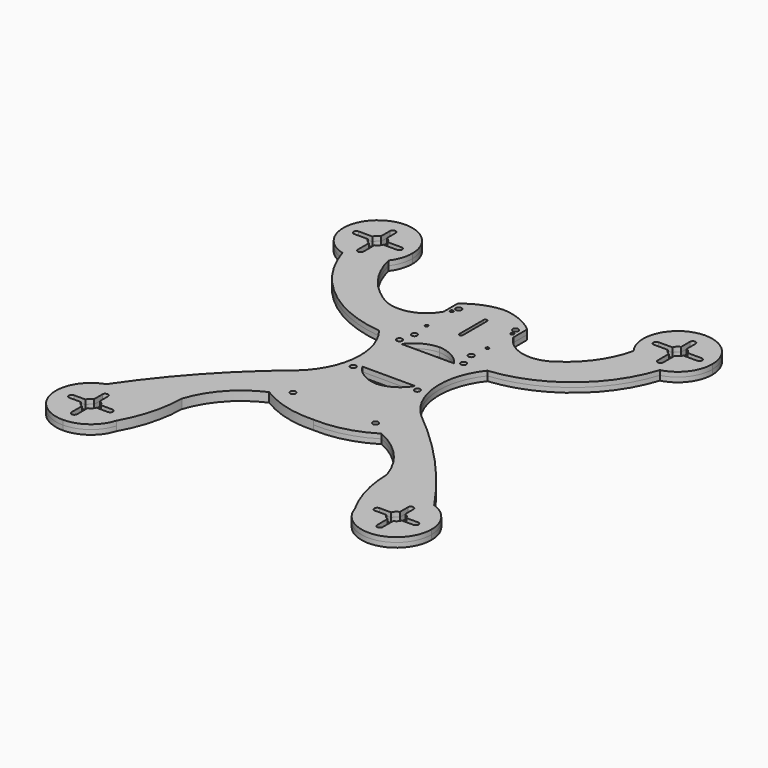
from build123d import *

# Parameters (mm, degrees)
F0_R     = 1.51
F0_R_2   = 1.5
F0_R_3   = 0.8286154485
F1_DEPTH = 2.5


# Not quite as in the source:
# - a feature names something its author has since deleted; it is built from what else it names


with BuildPart() as f1:
    # F0 (on Top) → F1 (new body, symmetric)
    with BuildSketch(Plane.XY):
        with BuildLine():
            Line((-30.1874730734, -52.384633545), (0, -52.384633545))
            Line((0, -52.384633545), (30.1874730734, -52.384633545))
            ThreePointArc((30.1874730734, -52.384633545), (45.5377526982, -63.4637920797), (55.0844569757, -79.8112468001))
            ThreePointArc((55.0844569757, -79.8112468001), (57.4877299486, -96.795391674), (64.006494816, -112.6617902157))
            ThreePointArc((64.006494816, -112.6617902157), (68.9048734281, -93.7156261949), (87.9887831434, -89.3848486541))
            ThreePointArc((87.9887831434, -89.3848486541), (62.7573722568, -57.4704416031), (33.2118480486, -29.5023263287))
            ThreePointArc((33.2118480486, -29.5023263287), (26.7242341229, -24.347436704), (20.0885272052, -19.384633545))
            Line((20.0885272052, -19.384633545), (21.4383106123, 19.6198565499))
            ThreePointArc((21.4383106123, 19.6198565499), (25.2461771825, 19.6733705963), (29.0445808108, 19.9469422451))
            ThreePointArc((29.0445808108, 19.9469422451), (63.9115542942, 34.3327431649), (85.1620762927, 65.494778124))
            ThreePointArc((85.1620762927, 65.494778124), (74.4508574846, 65.9052964442), (65.7591074705, 72.1784308553))
            ThreePointArc((65.7591074705, 72.1784308553), (58.8481462627, 56.5107805649), (46.674050137, 44.4680219955))
            ThreePointArc((46.674050137, 44.4680219955), (45.2140675367, 43.468299654), (43.6672608264, 42.60900753))
            ThreePointArc((43.6672608264, 42.60900753), (31.6040521188, 37.8807075534), (18.7, 36.713118625))
            Line((18.7, 36.713118625), (18.7, 50.3240376711))
            Line((18.7, 50.3240376711), (18.7, 59.615366455))
            ThreePointArc((18.7, 59.615366455), (9.9937787785, 65.0337535356), (0, 67.3319250345))
            ThreePointArc((0, 67.3319250345), (-9.9937787785, 65.0337535356), (-18.7, 59.615366455))
            Line((-18.7, 59.615366455), (-18.7, 50.3240376711))
            Line((-18.7, 50.3240376711), (-18.7, 36.713118625))
            ThreePointArc((-18.7, 36.713118625), (-31.6040521188, 37.8807075534), (-43.6672608264, 42.60900753))
            ThreePointArc((-43.6672608264, 42.60900753), (-45.2140675367, 43.468299654), (-46.674050137, 44.4680219955))
            ThreePointArc((-46.674050137, 44.4680219955), (-58.8481462627, 56.5107805649), (-65.7591074705, 72.1784308553))
            ThreePointArc((-65.7591074705, 72.1784308553), (-74.4508574846, 65.9052964442), (-85.1620762927, 65.494778124))
            ThreePointArc((-85.1620762927, 65.494778124), (-63.9115542942, 34.3327431649), (-29.0445808108, 19.9469422451))
            ThreePointArc((-29.0445808108, 19.9469422451), (-25.2461771825, 19.6733705963), (-21.4383106123, 19.6198565499))
            Line((-21.4383106123, 19.6198565499), (-20.0885272052, -19.384633545))
            ThreePointArc((-20.0885272052, -19.384633545), (-26.7242341229, -24.347436704), (-33.2118480486, -29.5023263287))
            ThreePointArc((-33.2118480486, -29.5023263287), (-62.7573722568, -57.4704416031), (-87.9887831434, -89.3848486541))
            ThreePointArc((-87.9887831434, -89.3848486541), (-71.0247151945, -91.9413319507), (-63.1980110774, -107.2075662893))
            ThreePointArc((-63.1980110774, -107.2075662893), (-63.4012302478, -109.9644759992), (-64.006494816, -112.6617902157))
            ThreePointArc((-64.006494816, -112.6617902157), (-57.4877299486, -96.795391674), (-55.0844569757, -79.8112468001))
            ThreePointArc((-55.0844569757, -79.8112468001), (-45.5377526982, -63.4637920797), (-30.1874730734, -52.384633545))
        make_face()
        with Locations((-22.1585966647, -46.4437194169)):
            Circle(F0_R, mode=Mode.SUBTRACT)
        with Locations((-17.2166451812, -12.1963914914)):
            Circle(F0_R_2, mode=Mode.SUBTRACT)
        with Locations((22.1585966647, -46.4437194169)):
            Circle(F0_R, mode=Mode.SUBTRACT)
        with BuildLine():
            Line((-14.1357257962, -9.8804375157), (0, -9.8804375157))
            Line((0, -9.8804375157), (14.1357257962, -9.8804375157))
            ThreePointArc((14.1357257962, -9.8804375157), (8.1506579233, -15.9532697198), (0, -18.4566881508))
            ThreePointArc((0, -18.4566881508), (-8.1506579233, -15.9532697198), (-14.1357257962, -9.8804375157))
        make_face(mode=Mode.SUBTRACT)
        with Locations((17.2166451812, -12.1963914914)):
            Circle(F0_R_2, mode=Mode.SUBTRACT)
        with BuildLine():
            ThreePointArc((-18.7, 18.5807666779), (-18.7166451812, 18.8036085086), (-18.7, 19.0264503392))
            ThreePointArc((-18.7, 19.0264503392), (-17.1049138701, 20.2994414251), (-15.7166451812, 18.8036085086))
            ThreePointArc((-15.7166451812, 18.8036085086), (-17.1049138701, 17.3077755921), (-18.7, 18.5807666779))
        make_face(mode=Mode.SUBTRACT)
        with Locations((-15.2508411556, 26.3805482537)):
            Circle(F0_R, mode=Mode.SUBTRACT)
        with Locations((-16.3033773307, 35.8986854553)):
            Circle(F0_R_3, mode=Mode.SUBTRACT)
        with BuildLine():
            ThreePointArc((-17.2290705489, 52.7536339848), (-16.3040705489, 53.6786339848), (-15.3790705489, 52.7536339848))
            ThreePointArc((-15.3790705489, 52.7536339848), (-16.3040705489, 51.8286339848), (-17.2290705489, 52.7536339848))
        make_face(mode=Mode.SUBTRACT)
        with Locations((-15.2508411556, 56.1236590147)):
            Circle(F0_R, mode=Mode.SUBTRACT)
        with BuildLine():
            ThreePointArc((-14.1357257962, 16.3518823683), (-7.9488995039, 21.8256144878), (0, 24.0736268461))
            ThreePointArc((0, 24.0736268461), (7.9488995039, 21.8256144878), (14.1357257962, 16.3518823683))
            Line((14.1357257962, 16.3518823683), (0, 16.3518823683))
            Line((0, 16.3518823683), (-14.1357257962, 16.3518823683))
        make_face(mode=Mode.SUBTRACT)
        with Locations((15.2508411556, 26.3805482537)):
            Circle(F0_R, mode=Mode.SUBTRACT)
        with BuildLine():
            ThreePointArc((18.7, 18.5807666779), (15.7166451812, 18.8036085086), (18.7, 19.0264503392))
            ThreePointArc((18.7, 19.0264503392), (18.7124780977, 18.9153398197), (18.7166451812, 18.8036085086))
            ThreePointArc((18.7166451812, 18.8036085086), (18.7124780977, 18.6918771974), (18.7, 18.5807666779))
        make_face(mode=Mode.SUBTRACT)
        with Locations((16.3033773307, 35.8986854553)):
            Circle(F0_R_3, mode=Mode.SUBTRACT)
        with BuildLine():
            ThreePointArc((0.925, 38.6986881495), (0.6540737726, 38.0446143769), (0, 37.7736881495))
            ThreePointArc((0, 37.7736881495), (-0.6540737726, 38.0446143769), (-0.925, 38.6986881495))
            Line((-0.925, 38.6986881495), (-0.925, 54.8593327403))
            ThreePointArc((-0.925, 54.8593327403), (-0.6540737726, 55.5134065129), (0, 55.7843327403))
            ThreePointArc((0, 55.7843327403), (0.6540737726, 55.5134065129), (0.925, 54.8593327403))
            Line((0.925, 54.8593327403), (0.925, 38.6986881495))
        make_face(mode=Mode.SUBTRACT)
        with Locations((15.2508411556, 56.1236590147)):
            Circle(F0_R, mode=Mode.SUBTRACT)
        with BuildLine():
            ThreePointArc((15.3790705489, 52.7536339848), (16.3040705489, 53.6786339848), (17.2290705489, 52.7536339848))
            ThreePointArc((17.2290705489, 52.7536339848), (16.3040705489, 51.8286339848), (15.3790705489, 52.7536339848))
        make_face(mode=Mode.SUBTRACT)
        with BuildLine():
            ThreePointArc((-82, -126.0095552119), (-70.7981133375, -122.3083120538), (-64.006494816, -112.6617902157))
            ThreePointArc((-64.006494816, -112.6617902157), (-63.4012302478, -109.9644759992), (-63.1980110774, -107.2075662893))
            ThreePointArc((-63.1980110774, -107.2075662893), (-71.0247151945, -91.9413319507), (-87.9887831434, -89.3848486541))
            ThreePointArc((-87.9887831434, -89.3848486541), (-100.5555561355, -110.241725802), (-82, -126.0095552119))
        make_face()
        with BuildLine():
            ThreePointArc((-80.5, -103.1137172447), (-78.917014434, -104.1245807233), (-77.9061509554, -105.7075662893))
            Line((-77.9061509554, -105.7075662893), (-71.66, -105.7075662893))
            ThreePointArc((-71.66, -105.7075662893), (-70.5993398282, -106.1469061175), (-70.16, -107.2075662893))
            ThreePointArc((-70.16, -107.2075662893), (-70.5993398282, -108.2682264611), (-71.66, -108.7075662893))
            Line((-71.66, -108.7075662893), (-77.9061509554, -108.7075662893))
            ThreePointArc((-77.9061509554, -108.7075662893), (-78.917014434, -110.2905518553), (-80.5, -111.3014153339))
            Line((-80.5, -111.3014153339), (-80.5, -118.2955773668))
            ThreePointArc((-80.5, -118.2955773668), (-82, -119.7955773668), (-83.5, -118.2955773668))
            Line((-83.5, -118.2955773668), (-83.5, -111.3014153339))
            ThreePointArc((-83.5, -111.3014153339), (-85.082985566, -110.2905518553), (-86.0938490446, -108.7075662893))
            Line((-86.0938490446, -108.7075662893), (-92.34, -108.7075662893))
            ThreePointArc((-92.34, -108.7075662893), (-93.84, -107.2075662893), (-92.34, -105.7075662893))
            Line((-92.34, -105.7075662893), (-86.0938490446, -105.7075662893))
            ThreePointArc((-86.0938490446, -105.7075662893), (-85.082985566, -104.1245807233), (-83.5, -103.1137172447))
            Line((-83.5, -103.1137172447), (-83.5, -97.6055773668))
            ThreePointArc((-83.5, -97.6055773668), (-82, -96.1055773668), (-80.5, -97.6055773668))
            Line((-80.5, -97.6055773668), (-80.5, -103.1137172447))
        make_face(mode=Mode.SUBTRACT)
        with BuildLine():
            ThreePointArc((87.9887831434, -89.3848486541), (68.9048734281, -93.7156261949), (64.006494816, -112.6617902157))
            ThreePointArc((64.006494816, -112.6617902157), (84.7569097099, -125.8063360415), (100.8019889226, -107.2075662893))
            ThreePointArc((100.8019889226, -107.2075662893), (97.2662343387, -96.2322814839), (87.9887831434, -89.3848486541))
        make_face()
        with BuildLine():
            Line((83.5, -111.3014153339), (83.5, -118.2955773668))
            ThreePointArc((83.5, -118.2955773668), (82, -119.7955773668), (80.5, -118.2955773668))
            Line((80.5, -118.2955773668), (80.5, -111.3014153339))
            ThreePointArc((80.5, -111.3014153339), (78.917014434, -110.2905518553), (77.9061509554, -108.7075662893))
            Line((77.9061509554, -108.7075662893), (71.66, -108.7075662893))
            ThreePointArc((71.66, -108.7075662893), (70.16, -107.2075662893), (71.66, -105.7075662893))
            Line((71.66, -105.7075662893), (77.9061509554, -105.7075662893))
            ThreePointArc((77.9061509554, -105.7075662893), (78.917014434, -104.1245807233), (80.5, -103.1137172447))
            Line((80.5, -103.1137172447), (80.5, -97.6055773668))
            ThreePointArc((80.5, -97.6055773668), (82, -96.1055773668), (83.5, -97.6055773668))
            Line((83.5, -97.6055773668), (83.5, -103.1137172447))
            ThreePointArc((83.5, -103.1137172447), (85.082985566, -104.1245807233), (86.0938490446, -105.7075662893))
            Line((86.0938490446, -105.7075662893), (92.34, -105.7075662893))
            ThreePointArc((92.34, -105.7075662893), (93.4006601718, -106.1469061175), (93.84, -107.2075662893))
            ThreePointArc((93.84, -107.2075662893), (93.4006601718, -108.2682264611), (92.34, -108.7075662893))
            Line((92.34, -108.7075662893), (86.0938490446, -108.7075662893))
            ThreePointArc((86.0938490446, -108.7075662893), (85.082985566, -110.2905518553), (83.5, -111.3014153339))
        make_face(mode=Mode.SUBTRACT)
        with BuildLine():
            ThreePointArc((-61.9557945169, 83.4250120531), (-67.3831058615, 96.5277007085), (-80.4857945169, 101.9550120531))
            ThreePointArc((-80.4857945169, 101.9550120531), (-98.8652413898, 85.7823055534), (-85.1620762927, 65.494778124))
            ThreePointArc((-85.1620762927, 65.494778124), (-74.4508574846, 65.9052964442), (-65.7591074705, 72.1784308553))
            ThreePointArc((-65.7591074705, 72.1784308553), (-62.932355951, 77.4888774088), (-61.9557945169, 83.4250120531))
        make_face()
        with BuildLine():
            ThreePointArc((-78.9857945169, 87.5188610977), (-77.4028089509, 86.507997619), (-76.3919454723, 84.9250120531))
            Line((-76.3919454723, 84.9250120531), (-68.9257945169, 84.9250120531))
            ThreePointArc((-68.9257945169, 84.9250120531), (-67.8651343451, 84.4856722249), (-67.4257945169, 83.4250120531))
            ThreePointArc((-67.4257945169, 83.4250120531), (-67.8651343451, 82.3643518813), (-68.9257945169, 81.9250120531))
            Line((-68.9257945169, 81.9250120531), (-76.3919454723, 81.9250120531))
            ThreePointArc((-76.3919454723, 81.9250120531), (-77.4028089509, 80.3420264871), (-78.9857945169, 79.3311630085))
            Line((-78.9857945169, 79.3311630085), (-78.9857945169, 71.8650120531))
            ThreePointArc((-78.9857945169, 71.8650120531), (-80.4857945169, 70.3650120531), (-81.9857945169, 71.8650120531))
            Line((-81.9857945169, 71.8650120531), (-81.9857945169, 79.3311630085))
            ThreePointArc((-81.9857945169, 79.3311630085), (-83.5687800828, 80.3420264871), (-84.5796435615, 81.9250120531))
            Line((-84.5796435615, 81.9250120531), (-92.0457945169, 81.9250120531))
            ThreePointArc((-92.0457945169, 81.9250120531), (-93.5457945169, 83.4250120531), (-92.0457945169, 84.9250120531))
            Line((-92.0457945169, 84.9250120531), (-84.5796435615, 84.9250120531))
            ThreePointArc((-84.5796435615, 84.9250120531), (-83.5687800828, 86.507997619), (-81.9857945169, 87.5188610977))
            Line((-81.9857945169, 87.5188610977), (-81.9857945169, 93.4850120531))
            ThreePointArc((-81.9857945169, 93.4850120531), (-80.4857945169, 94.9850120531), (-78.9857945169, 93.4850120531))
            Line((-78.9857945169, 93.4850120531), (-78.9857945169, 87.5188610977))
        make_face(mode=Mode.SUBTRACT)
        with BuildLine():
            ThreePointArc((65.7591074705, 72.1784308553), (74.4508574846, 65.9052964442), (85.1620762927, 65.494778124))
            ThreePointArc((85.1620762927, 65.494778124), (95.1488842545, 72.0956387541), (99.0157945169, 83.4250120531))
            ThreePointArc((99.0157945169, 83.4250120531), (74.5496598725, 100.9784506189), (65.7591074705, 72.1784308553))
        make_face()
        with BuildLine():
            ThreePointArc((81.9857945169, 87.5188610977), (83.5687800828, 86.507997619), (84.5796435615, 84.9250120531))
            Line((84.5796435615, 84.9250120531), (92.0457945169, 84.9250120531))
            ThreePointArc((92.0457945169, 84.9250120531), (93.1064546886, 84.4856722249), (93.5457945169, 83.4250120531))
            ThreePointArc((93.5457945169, 83.4250120531), (93.1064546886, 82.3643518813), (92.0457945169, 81.9250120531))
            Line((92.0457945169, 81.9250120531), (84.5796435615, 81.9250120531))
            ThreePointArc((84.5796435615, 81.9250120531), (83.5687800828, 80.3420264871), (81.9857945169, 79.3311630085))
            Line((81.9857945169, 79.3311630085), (81.9857945169, 71.8650120531))
            ThreePointArc((81.9857945169, 71.8650120531), (80.4857945169, 70.3650120531), (78.9857945169, 71.8650120531))
            Line((78.9857945169, 71.8650120531), (78.9857945169, 79.3311630085))
            ThreePointArc((78.9857945169, 79.3311630085), (77.4028089509, 80.3420264871), (76.3919454723, 81.9250120531))
            Line((76.3919454723, 81.9250120531), (68.9257945169, 81.9250120531))
            ThreePointArc((68.9257945169, 81.9250120531), (67.4257945169, 83.4250120531), (68.9257945169, 84.9250120531))
            Line((68.9257945169, 84.9250120531), (76.3919454723, 84.9250120531))
            ThreePointArc((76.3919454723, 84.9250120531), (77.4028089509, 86.507997619), (78.9857945169, 87.5188610977))
            Line((78.9857945169, 87.5188610977), (78.9857945169, 93.4850120531))
            ThreePointArc((78.9857945169, 93.4850120531), (80.4857945169, 94.9850120531), (81.9857945169, 93.4850120531))
            Line((81.9857945169, 93.4850120531), (81.9857945169, 87.5188610977))
        make_face(mode=Mode.SUBTRACT)
        with BuildLine():
            Line((30.1874730734, -52.384633545), (0, -52.384633545))
            Line((0, -52.384633545), (-30.1874730734, -52.384633545))
            ThreePointArc((-30.1874730734, -52.384633545), (-15.6968009353, -58.6423760096), (0, -60.3004954755))
            ThreePointArc((0, -60.3004954755), (15.6968009353, -58.6423760096), (30.1874730734, -52.384633545))
        make_face()
        with BuildLine():
            ThreePointArc((-29.0445808108, 19.9469422451), (-21.3446813988, -5.6021854639), (-33.2118480486, -29.5023263287))
            ThreePointArc((-33.2118480486, -29.5023263287), (-26.7242341229, -24.347436704), (-20.0885272052, -19.384633545))
            Line((-20.0885272052, -19.384633545), (-21.4383106123, 19.6198565499))
            ThreePointArc((-21.4383106123, 19.6198565499), (-25.2461771825, 19.6733705963), (-29.0445808108, 19.9469422451))
        make_face()
        with BuildLine():
            ThreePointArc((20.0885272052, -19.384633545), (26.7242341229, -24.347436704), (33.2118480486, -29.5023263287))
            ThreePointArc((33.2118480486, -29.5023263287), (21.3446813988, -5.6021854639), (29.0445808108, 19.9469422451))
            ThreePointArc((29.0445808108, 19.9469422451), (25.2461771825, 19.6733705963), (21.4383106123, 19.6198565499))
            Line((21.4383106123, 19.6198565499), (20.0885272052, -19.384633545))
        make_face()
        with BuildLine():
            ThreePointArc((-18.7, 50.3240376711), (-29.6426565817, 41.4796469988), (-43.6672608264, 42.60900753))
            ThreePointArc((-43.6672608264, 42.60900753), (-31.6040521188, 37.8807075534), (-18.7, 36.713118625))
            Line((-18.7, 36.713118625), (-18.7, 50.3240376711))
        make_face()
        with BuildLine():
            ThreePointArc((18.7, 36.713118625), (31.6040521188, 37.8807075534), (43.6672608264, 42.60900753))
            ThreePointArc((43.6672608264, 42.60900753), (29.6426565817, 41.4796469988), (18.7, 50.3240376711))
            Line((18.7, 50.3240376711), (18.7, 36.713118625))
        make_face()
        with BuildLine():
            ThreePointArc((-43.6672608264, 42.60900753), (-45.1885647911, 43.5095480596), (-46.674050137, 44.4680219955))
            ThreePointArc((-46.674050137, 44.4680219955), (-45.2140675367, 43.468299654), (-43.6672608264, 42.60900753))
        make_face()
        with BuildLine():
            Line((-18.7, 18.5807666779), (-18.7, 19.0264503392))
            ThreePointArc((-18.7, 19.0264503392), (-18.7166451812, 18.8036085086), (-18.7, 18.5807666779))
        make_face()
    extrude(amount=F1_DEPTH, both=True)


solid = f1.part
